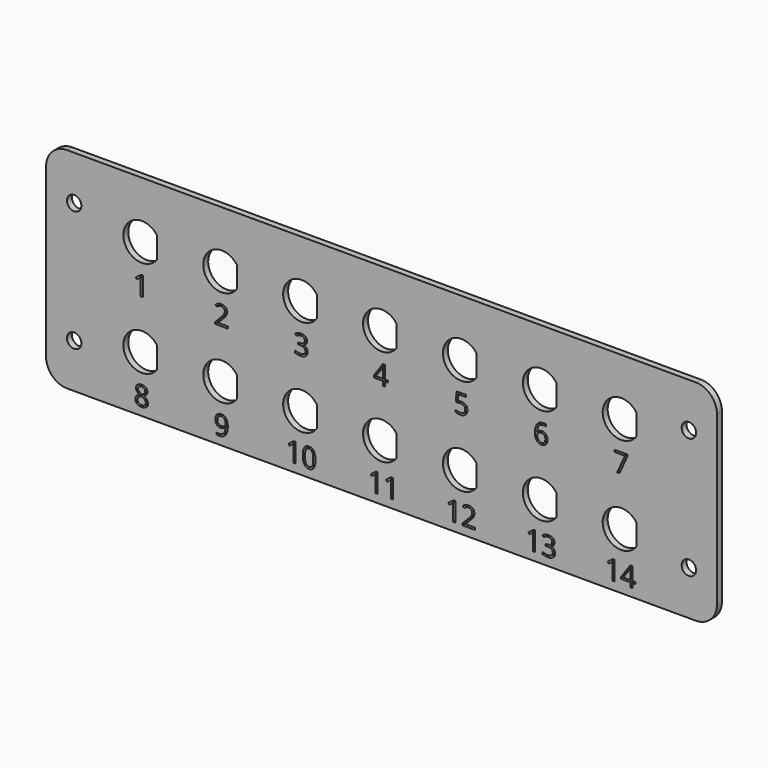
from build123d import *

# Parameters (mm, degrees)
F1_DEPTH     = 1.6256
F2_R         = 1.8923
F3_DEPTH     = 1.6266
F5_DEPTH     = 1.6266
F6_TEXT_SIZE = 7.0555555556
F7_DEPTH     = 1.27
F8_DEPTH     = 1.27


# Not quite as in the source:
# - Text() gives the source's letters only with a copy of the font that has no kerning and outlines rounded to 1/6400 em; it was checked with that copy


with BuildPart() as f1:
    # F0 (on Front) → F1 (new body)
    with BuildSketch(Plane.XZ):
        with BuildLine():
            Line((170.434, 55.0418), (5.5372, 55.0418))
            ThreePointArc((5.5372, 55.0418), (1.6218083312, 53.4199916688), (0, 49.5046))
            Line((0, 49.5046), (0, 5.5372))
            ThreePointArc((0, 5.5372), (1.6218083312, 1.6218083312), (5.5372, 0))
            Line((5.5372, 0), (170.434, 0))
            ThreePointArc((170.434, 0), (174.3493916688, 1.6218083312), (175.9712, 5.5372))
            Line((175.9712, 5.5372), (175.9712, 49.5046))
            ThreePointArc((175.9712, 49.5046), (174.3493916688, 53.4199916688), (170.434, 55.0418))
        make_face()
    extrude(amount=F1_DEPTH)

    # F2 (on face) → F3 (cut, through all)
    with BuildSketch(Plane.XZ.offset(1.6256)):
        with Locations((7.366, 43.3959)):
            Circle(F2_R)
        with Locations((7.366, 11.6459)):
            Circle(F2_R)
        with Locations((168.6052, 43.3959)):
            Circle(F2_R)
        with Locations((168.6052, 11.6459)):
            Circle(F2_R)
    extrude(amount=-F3_DEPTH, mode=Mode.SUBTRACT)

    # F4 (on face) → F5 (cut, through all)
    with BuildSketch(Plane.XZ.offset(1.6256)):
        with BuildLine():
            Line((29.1084, 37.458015073), (29.1084, 42.983784927))
            ThreePointArc((29.1084, 42.983784927), (20.2692, 40.2209), (29.1084, 37.458015073))
        make_face()
        with BuildLine():
            Line((29.1084, 12.058015073), (29.1084, 17.583784927))
            ThreePointArc((29.1084, 17.583784927), (20.2692, 14.8209), (29.1084, 12.058015073))
        make_face()
        with BuildLine():
            Line((50.0634, 37.458015073), (50.0634, 42.983784927))
            ThreePointArc((50.0634, 42.983784927), (41.2242, 40.2209), (50.0634, 37.458015073))
        make_face()
        with BuildLine():
            Line((50.0634, 12.058015073), (50.0634, 17.583784927))
            ThreePointArc((50.0634, 17.583784927), (41.2242, 14.8209), (50.0634, 12.058015073))
        make_face()
        with BuildLine():
            Line((71.0184, 37.458015073), (71.0184, 42.983784927))
            ThreePointArc((71.0184, 42.983784927), (62.1792, 40.2209), (71.0184, 37.458015073))
        make_face()
        with BuildLine():
            Line((71.0184, 12.058015073), (71.0184, 17.583784927))
            ThreePointArc((71.0184, 17.583784927), (62.1792, 14.8209), (71.0184, 12.058015073))
        make_face()
        with BuildLine():
            Line((91.9734, 37.458015073), (91.9734, 42.983784927))
            ThreePointArc((91.9734, 42.983784927), (83.1342, 40.2209), (91.9734, 37.458015073))
        make_face()
        with BuildLine():
            Line((91.9734, 12.058015073), (91.9734, 17.583784927))
            ThreePointArc((91.9734, 17.583784927), (83.1342, 14.8209), (91.9734, 12.058015073))
        make_face()
        with BuildLine():
            Line((112.9284, 37.458015073), (112.9284, 42.983784927))
            ThreePointArc((112.9284, 42.983784927), (104.0892, 40.2209), (112.9284, 37.458015073))
        make_face()
        with BuildLine():
            Line((112.9284, 12.058015073), (112.9284, 17.583784927))
            ThreePointArc((112.9284, 17.583784927), (104.0892, 14.8209), (112.9284, 12.058015073))
        make_face()
        with BuildLine():
            Line((133.8834, 37.458015073), (133.8834, 42.983784927))
            ThreePointArc((133.8834, 42.983784927), (125.0442, 40.2209), (133.8834, 37.458015073))
        make_face()
        with BuildLine():
            Line((133.8834, 12.058015073), (133.8834, 17.583784927))
            ThreePointArc((133.8834, 17.583784927), (125.0442, 14.8209), (133.8834, 12.058015073))
        make_face()
        with BuildLine():
            Line((154.8384, 37.458015073), (154.8384, 42.983784927))
            ThreePointArc((154.8384, 42.983784927), (145.9992, 40.2209), (154.8384, 37.458015073))
        make_face()
        with BuildLine():
            Line((154.8384, 12.058015073), (154.8384, 17.583784927))
            ThreePointArc((154.8384, 17.583784927), (145.9992, 14.8209), (154.8384, 12.058015073))
        make_face()
    extrude(amount=-F5_DEPTH, mode=Mode.SUBTRACT)

    # F6 (on face) → F7 (cut)
    with BuildSketch(Plane.XZ.offset(1.6256)):
        with Locations((22.9102045705, 27.5209)):
            Text('1', F6_TEXT_SIZE, font='Open Sans', text_align=(TextAlign.LEFT, TextAlign.BOTTOM))
        with Locations((44.0190157986, 27.5209)):
            Text('2', F6_TEXT_SIZE, font='Open Sans', text_align=(TextAlign.LEFT, TextAlign.BOTTOM))
        with Locations((64.9916546875, 27.5209)):
            Text('3', F6_TEXT_SIZE, font='Open Sans', text_align=(TextAlign.LEFT, TextAlign.BOTTOM))
        with Locations((85.8105045139, 27.5209)):
            Text('4', F6_TEXT_SIZE, font='Open Sans', text_align=(TextAlign.LEFT, TextAlign.BOTTOM))
        with Locations((106.8977961806, 27.5209)):
            Text('5', F6_TEXT_SIZE, font='Open Sans', text_align=(TextAlign.LEFT, TextAlign.BOTTOM))
        with Locations((127.821928125, 27.5209)):
            Text('6', F6_TEXT_SIZE, font='Open Sans', text_align=(TextAlign.LEFT, TextAlign.BOTTOM))
        with Locations((148.7840939236, 27.5209)):
            Text('7', F6_TEXT_SIZE, font='Open Sans', text_align=(TextAlign.LEFT, TextAlign.BOTTOM))
        with Locations((23.0574012153, 2.1209)):
            Text('8', F6_TEXT_SIZE, font='Open Sans', text_align=(TextAlign.LEFT, TextAlign.BOTTOM))
        with Locations((44.0190157986, 2.1209)):
            Text('9', F6_TEXT_SIZE, font='Open Sans', text_align=(TextAlign.LEFT, TextAlign.BOTTOM))
        with Locations((62.9433387153, 2.1209)):
            Text('10', F6_TEXT_SIZE, font='Open Sans', text_align=(TextAlign.LEFT, TextAlign.BOTTOM))
        with Locations((84.5085340278, 2.1209)):
            Text('11', F6_TEXT_SIZE, font='Open Sans', text_align=(TextAlign.LEFT, TextAlign.BOTTOM))
        with Locations((104.8671190972, 2.1209)):
            Text('12', F6_TEXT_SIZE, font='Open Sans', text_align=(TextAlign.LEFT, TextAlign.BOTTOM))
        with Locations((125.8397579861, 2.1209)):
            Text('13', F6_TEXT_SIZE, font='Open Sans', text_align=(TextAlign.LEFT, TextAlign.BOTTOM))
        with Locations((146.6586078125, 2.1209)):
            Text('14', F6_TEXT_SIZE, font='Open Sans', text_align=(TextAlign.LEFT, TextAlign.BOTTOM))
    extrude(amount=-F7_DEPTH, mode=Mode.SUBTRACT)

    # F6 (on face) → F8 (cut)
    with BuildSketch(Plane.XZ.offset(1.6256)):
        with Locations((22.9102045705, 27.5209)):
            Text('1', F6_TEXT_SIZE, font='Open Sans', text_align=(TextAlign.LEFT, TextAlign.BOTTOM))
        with Locations((44.0190157986, 27.5209)):
            Text('2', F6_TEXT_SIZE, font='Open Sans', text_align=(TextAlign.LEFT, TextAlign.BOTTOM))
        with Locations((64.9916546875, 27.5209)):
            Text('3', F6_TEXT_SIZE, font='Open Sans', text_align=(TextAlign.LEFT, TextAlign.BOTTOM))
        with Locations((85.8105045139, 27.5209)):
            Text('4', F6_TEXT_SIZE, font='Open Sans', text_align=(TextAlign.LEFT, TextAlign.BOTTOM))
        with Locations((106.8977961806, 27.5209)):
            Text('5', F6_TEXT_SIZE, font='Open Sans', text_align=(TextAlign.LEFT, TextAlign.BOTTOM))
        with Locations((127.821928125, 27.5209)):
            Text('6', F6_TEXT_SIZE, font='Open Sans', text_align=(TextAlign.LEFT, TextAlign.BOTTOM))
        with Locations((148.7840939236, 27.5209)):
            Text('7', F6_TEXT_SIZE, font='Open Sans', text_align=(TextAlign.LEFT, TextAlign.BOTTOM))
        with Locations((23.0574012153, 2.1209)):
            Text('8', F6_TEXT_SIZE, font='Open Sans', text_align=(TextAlign.LEFT, TextAlign.BOTTOM))
        with Locations((44.0190157986, 2.1209)):
            Text('9', F6_TEXT_SIZE, font='Open Sans', text_align=(TextAlign.LEFT, TextAlign.BOTTOM))
        with Locations((62.9433387153, 2.1209)):
            Text('10', F6_TEXT_SIZE, font='Open Sans', text_align=(TextAlign.LEFT, TextAlign.BOTTOM))
        with Locations((84.5085340278, 2.1209)):
            Text('11', F6_TEXT_SIZE, font='Open Sans', text_align=(TextAlign.LEFT, TextAlign.BOTTOM))
        with Locations((104.8671190972, 2.1209)):
            Text('12', F6_TEXT_SIZE, font='Open Sans', text_align=(TextAlign.LEFT, TextAlign.BOTTOM))
        with Locations((125.8397579861, 2.1209)):
            Text('13', F6_TEXT_SIZE, font='Open Sans', text_align=(TextAlign.LEFT, TextAlign.BOTTOM))
        with Locations((146.6586078125, 2.1209)):
            Text('14', F6_TEXT_SIZE, font='Open Sans', text_align=(TextAlign.LEFT, TextAlign.BOTTOM))
    extrude(amount=-F8_DEPTH, mode=Mode.SUBTRACT)


solid = f1.part
